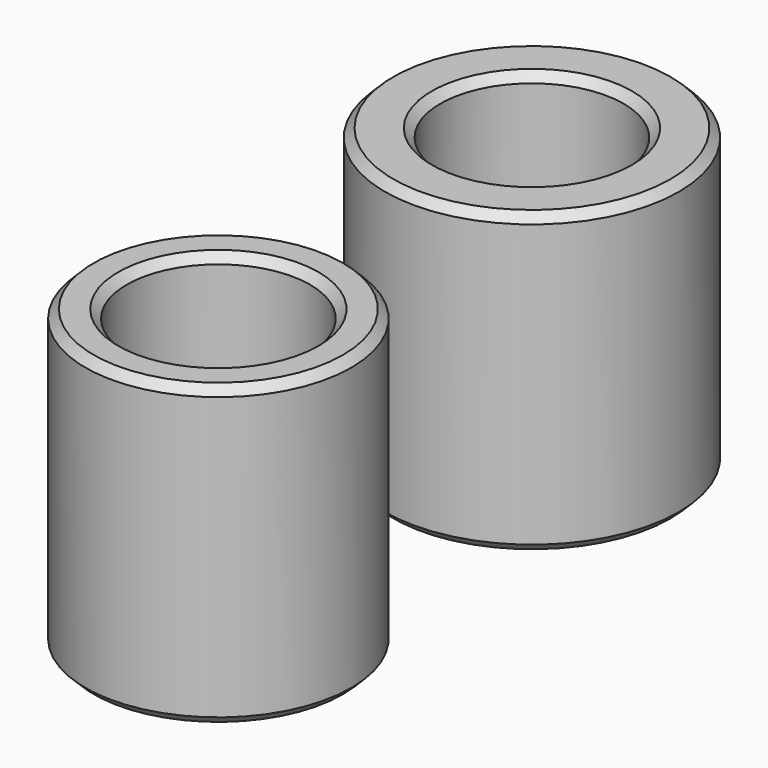
from build123d import *

# Parameters (mm, degrees)
F0_R      = 4.75
F0_R_2    = 3.275
F1_DEPTH  = 10.668
F0_R_3    = 5.25
F2_SIZE   = 0.3
F2_2_SIZE = 0.3


with BuildPart() as f1:
    # F0 (on Top) → F1 (new body)
    with BuildSketch(Plane.XY):
        with Locations((0, -14)):
            Circle(F0_R)
        with Locations((0, -14)):
            Circle(F0_R_2, mode=Mode.SUBTRACT)
    extrude(amount=F1_DEPTH)

    # F2
    f2_edges = [f1.edges().sort_by_distance(p)[0] for p in [
        (-3.275, -14, 10.668),
        (-3.275, -14, 0),
        (-4.75, -14, 0),
        (-4.75, -14, 10.668),
    ]]
    chamfer(f2_edges, length=F2_SIZE)


with BuildPart() as f1b:
    # F0 (on Top) → F1, piece 2 (new body)
    with BuildSketch(Plane.XY):
        Circle(F0_R_3)
        Circle(F0_R_2, mode=Mode.SUBTRACT)
    extrude(amount=F1_DEPTH)

    # F2#2
    f2_2_edges = [f1b.edges().sort_by_distance(p)[0] for p in [
        (-3.275, 0, 10.668),
        (-3.275, 0, 0),
        (-5.25, 0, 0),
        (-5.25, 0, 10.668),
    ]]
    chamfer(f2_2_edges, length=F2_2_SIZE)


solid = Compound([f1.part, f1b.part])
